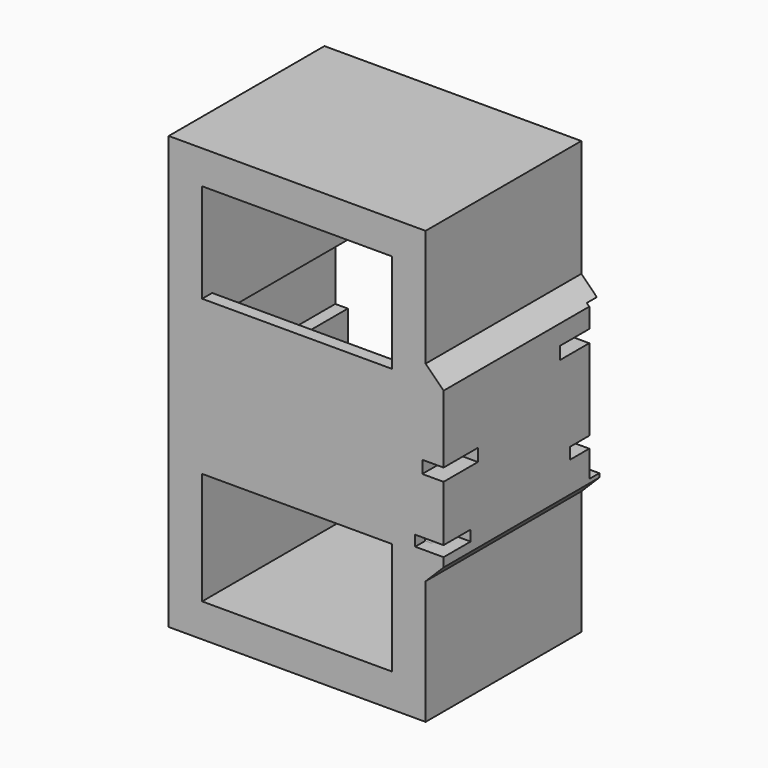
from build123d import *

# Parameters (mm, degrees)
F0_W        = 615
F0_H        = 1035
F1_DEPTH    = 436
F2_W        = 383.7750256062
F2_H        = 30
F2_W_2      = 88.2078781724
F3_DEPTH    = 10
F4_W        = 436
F4_H        = 368.6535954475
F5_DEPTH    = 43
F6_T4_DEPTH = 436
F6_T9_DEPTH = 436
F7_W        = 102.6465103626
F7_H        = 30
F7_W_2      = 88.2078781724
F8_DEPTH    = 51
F9_W        = 30
F9_H        = 30
F10_DEPTH   = 55
F11_W       = 30
F11_H       = 30
F12_DEPTH   = 100
F14_DEPTH   = 30
F15_W       = 53
F15_H       = 27.2612595558
F16_DEPTH   = 57
F17_W       = 67.928535223
F17_H       = 25.3568291664
F18_DEPTH   = 81
F20_DEPTH   = 30
F22_DEPTH   = 25


# Not quite as in the source:
# - a fillet or chamfer that OpenCascade refuses, or shapes differently, is made with other operations: its cross-section is extruded or revolved along the edge and cut away or added


with BuildPart() as f1:
    # F0 (on Front) → F1 (new body)
    with BuildSketch(Plane.XZ):
        with Locations((0, 517.5)):
            Rectangle(F0_W, F0_H)
        Polygon((227.5, 80), (-227.5, 80), (-227.5, 360), (-257.5, 360), (-257.5, 440), (-227.5, 440), (-227.5, 520), (-257.5, 520), (-257.5, 665), (-227.5, 665), (-227.5, 955), (227.5, 955), (227.5, 665), (267.5, 665), (297.5, 665), (297.5, 635), (267.5, 635), (267.5, 550), (297.5, 550), (297.5, 520), (267.5, 520), (227.5, 520), (227.5, 440), (297.5, 440), (297.5, 360), (227.5, 360), align=None, mode=Mode.SUBTRACT)
    extrude(amount=F1_DEPTH)

    # F2 (on face) → F3 (cut, through all)
    with BuildSketch(Plane.YZ.offset(307.5)):
        with Locations((-191.8875128031, 535)):
            Rectangle(F2_W, F2_H)
        with Locations((-44.1039390862, 650)):
            Rectangle(F2_W_2, F2_H)
    extrude(amount=-F3_DEPTH, mode=Mode.SUBTRACT)

    # F4 (on face) → F5 (join)
    with BuildSketch(Plane.YZ.offset(307.5)):
        with Locations((-218, 525.7607400417)):
            Rectangle(F4_W, F4_H)
    extrude(amount=F5_DEPTH)

    # F6: chamfer of 45 on 2 edges, made by hand


with BuildPart() as f6_tool2:
    # F6_s3 → F6_t4 (new body)
    with BuildSketch(Plane.XZ):
        Polygon((307.5, 755.0875377655), (352.5, 710.0875377655), (307.5, 710.0875377655), align=None)
    extrude(amount=F6_T4_DEPTH)

    split(bisect_by=Plane.YZ.offset(350.5), keep=Keep.BOTTOM)


with BuildPart() as f1_1:
    add(f1.part)

    # F6_t1: union F6_tool2
    add(f6_tool2.part)


with BuildPart() as f6_tool7:
    # F6_s8 → F6_t9 (new body)
    with BuildSketch(Plane.XZ.offset(436)):
        Polygon((307.5, 296.433942318), (352.5, 341.433942318), (307.5, 341.433942318), align=None)
    extrude(amount=-F6_T9_DEPTH)

    split(bisect_by=Plane.YZ.offset(350.5), keep=Keep.BOTTOM)


with BuildPart() as f1_2:
    add(f1_1.part)

    # F6_t6: union F6_tool7
    add(f6_tool7.part)

    # F7 (on face) → F8 (cut)
    with BuildSketch(Plane.YZ.offset(350.5)):
        with Locations((-384.6767448187, 535)):
            Rectangle(F7_W, F7_H)
        with Locations((-44.1039390862, 650)):
            Rectangle(F7_W_2, F7_H)
    extrude(amount=-F8_DEPTH, mode=Mode.SUBTRACT)

    # F9 (on face) → F10 (join)
    with BuildSketch(Plane.XZ.offset(436)):
        with Locations((282.5, 535)):
            Rectangle(F9_W, F9_H)
    extrude(amount=-F10_DEPTH)

    # F11 (on face) → F12 (join)
    with BuildSketch(Plane.XZ.offset(436)):
        with Locations((282.5, 650)):
            Rectangle(F11_W, F11_H)
    extrude(amount=-F12_DEPTH)

    # F13 (on face) → F14 (join)
    with BuildSketch(Plane.XZ.offset(436)):
        Polygon((227.5, 665), (227.5, 717.9152965546), (-227.5, 717.9152965546), (-227.5, 665), (-257.5, 665), (-257.5, 520), (-227.5, 520), (-227.5, 440), (-257.5, 440), (-257.5, 360), (-227.5, 360), (-227.5, 348.8455712795), (227.5, 348.8455712795), (227.5, 360), (297.5, 360), (297.5, 440), (227.5, 440), (227.5, 520), (267.5, 520), (267.5, 665), align=None)
    extrude(amount=-F14_DEPTH)

    # F15 (on face) → F16 (cut)
    with BuildSketch(Plane(origin=(0, 0, 0), x_dir=(-1, 0, 0), z_dir=(0, 1, 0))):
        with Locations((-324, 426.3693702221)):
            Rectangle(F15_W, F15_H)
    extrude(amount=-F16_DEPTH, mode=Mode.SUBTRACT)

    # F17 (on face) → F18 (cut)
    with BuildSketch(Plane.XZ.offset(436)):
        with Locations((316.5357323885, 373.8530278206)):
            Rectangle(F17_W, F17_H)
    extrude(amount=-F18_DEPTH, mode=Mode.SUBTRACT)

    # F19 (on face) → F20 (join)
    with BuildSketch(Plane(origin=(0, 0, 0), x_dir=(-1, 0, 0), z_dir=(0, 1, 0))):
        Polygon((307.5, 0), (307.5, 348.8455712795), (227.5, 348.8455712795), (227.5, 80), (-227.5, 80), (-227.5, 348.8455712795), (-350.5, 348.8455712795), (-350.5, 339.433942318), (-307.5, 296.433942318), (-307.5, 0), align=None)
        Polygon((-359.9116289616, 348.8455712795), (-350.5, 339.433942318), (-350.5, 348.8455712795), align=None)
        Polygon((-344.6722412109, 717.9152965546), (-227.5, 717.9152965546), (-227.5, 955), (227.5, 955), (227.5, 717.9152965546), (307.5, 717.9152965546), (307.5, 1035), (-307.5, 1035), (-307.5, 755.0875377655), align=None)
    extrude(amount=F20_DEPTH)

    # F21 (on face) → F22 (cut)
    with BuildSketch(Plane.YZ.offset(350.5)):
        Polygon((52.2877275944, 373.7032711506), (0, 373.7032711506), (0, 348.8455712795), (0, 339.433942318), (-23.2749842107, 339.433942318), (-23.2749842107, 317.8108334541), (52.2877275944, 317.8108334541), align=None)
    extrude(amount=F22_DEPTH, mode=Mode.SUBTRACT)


solid = f1_2.part
